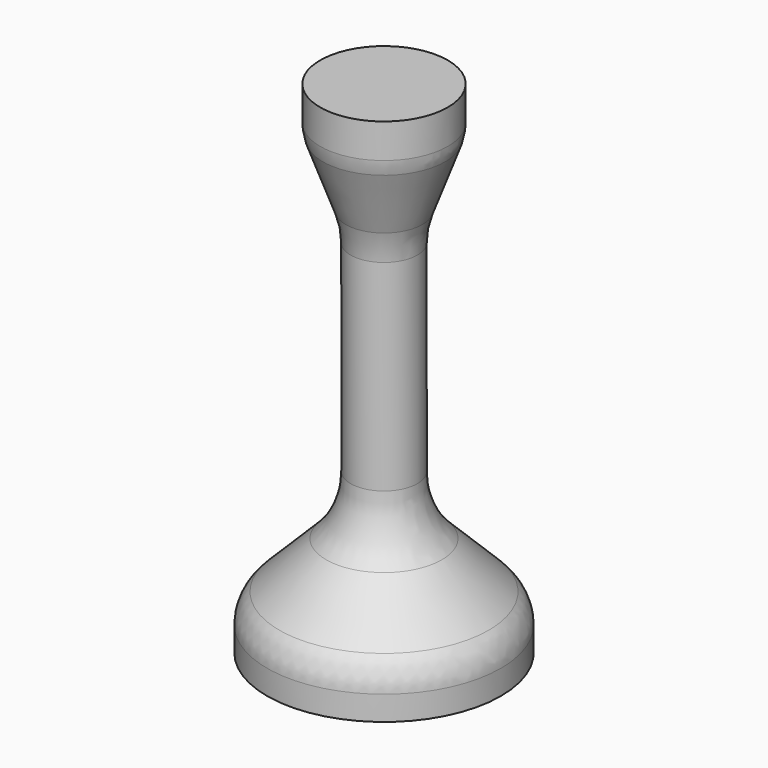
from build123d import *

# Parameters (mm, degrees)
F2_R = 10
F3_R = 5


with BuildPart() as f1:
    # F0 (on Front) → F1 (revolve)
    with BuildSketch(Plane.XZ):
        Polygon((7.6397023427, 30), (0, 30), (0, -30), (7.6397023427, -30), (14, -30), (14, -25), (4, -15), (4, 0), (4, 15), (7.6397023427, 25), align=None)
    revolve(axis=Axis((0, 0, 0), (0, 0, -1)))

    # F2
    f2_edges = [f1.edges().sort_by_distance(p)[0] for p in [
        (-4, 0, 15),
        (-4, 0, -15),
    ]]
    fillet(f2_edges, radius=F2_R)

    # F3
    f3_edges = [f1.edges().sort_by_distance(p)[0] for p in [
        (-7.639702, 0, 25),
        (-14, 0, -25),
    ]]
    fillet(f3_edges, radius=F3_R)


solid = f1.part
